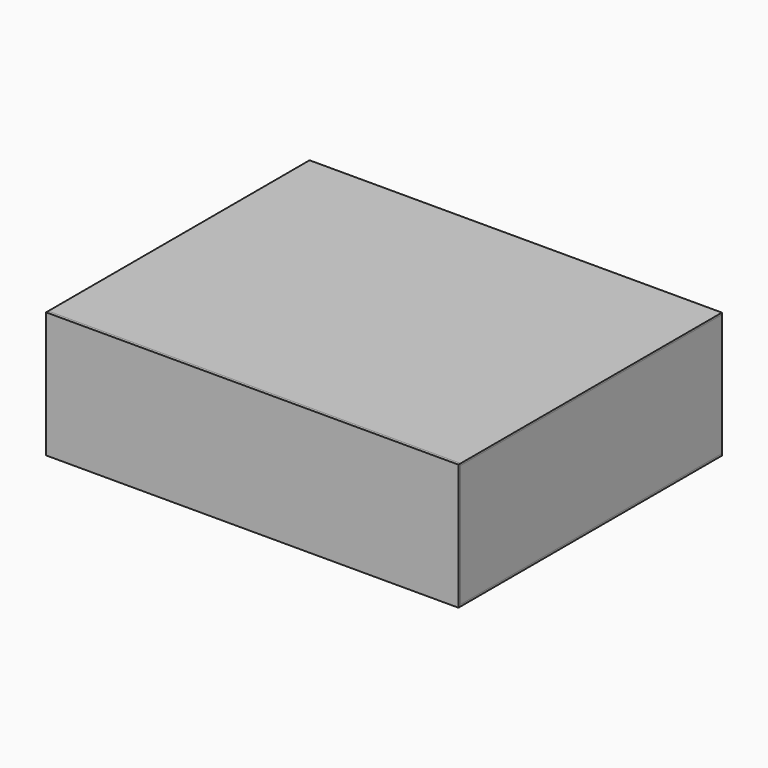
from build123d import *

# Parameters (mm, degrees)
F4_W      = 442
F4_H      = 350
F7_DEPTH  = 2
F0_W      = 442
F0_H      = 350
F8_DEPTH  = 2
F9_W      = 442
F9_H      = 131
F10_DEPTH = 2
F11_W     = 348
F11_H     = 131
F12_DEPTH = 2
F13_W     = 348
F13_H     = 131
F14_DEPTH = 2
F15_W     = 13
F15_H     = 131
F15_R     = 2
F16_DEPTH = 2
F17_W     = 442
F17_H     = 135
F18_DEPTH = 3


with BuildPart() as f7:
    # F4 (on offset) → F7 (new body)
    with BuildSketch(Plane.XY.offset(133)):
        Rectangle(F4_W, F4_H)
    extrude(amount=F7_DEPTH)


with BuildPart() as f8:
    # F0 (on Top) → F8 (new body)
    with BuildSketch(Plane.XY):
        Rectangle(F0_W, F0_H)
    extrude(amount=F8_DEPTH)


with BuildPart() as f10:
    # F9 (on offset) → F10 (new body)
    with BuildSketch(Plane.XZ.offset(-175)):
        with Locations((0, 67.5)):
            Rectangle(F9_W, F9_H)
    extrude(amount=F10_DEPTH)

    # F11 (on offset) → F12 (join)
    with BuildSketch(Plane.YZ.offset(-221)):
        with Locations((-1, 67.5)):
            Rectangle(F11_W, F11_H)
    extrude(amount=F12_DEPTH)

    # F13 (on offset) → F14 (join)
    with BuildSketch(Plane.YZ.offset(221)):
        with Locations((-1, 67.5)):
            Rectangle(F13_W, F13_H)
    extrude(amount=-F14_DEPTH)

    # F15 (on offset) → F16 (join)
    with BuildSketch(Plane.XZ.offset(175)):
        with Locations((-212.5, 67.5)):
            Rectangle(F15_W, F15_H)
        with Locations((-211, 35)):
            Circle(F15_R, mode=Mode.SUBTRACT)
        with Locations((-211, 100)):
            Circle(F15_R, mode=Mode.SUBTRACT)
        with Locations((212.5, 67.5)):
            Rectangle(F15_W, F15_H)
        with Locations((211, 35)):
            Circle(F15_R, mode=Mode.SUBTRACT)
        with Locations((211, 100)):
            Circle(F15_R, mode=Mode.SUBTRACT)
    extrude(amount=-F16_DEPTH)


with BuildPart() as f18:
    # F17 (on offset) → F18 (new body)
    with BuildSketch(Plane.XZ.offset(175)):
        with Locations((0, 67.5)):
            Rectangle(F17_W, F17_H)
    extrude(amount=F18_DEPTH)


solid = Compound([f7.part, f8.part, f10.part, f18.part])
